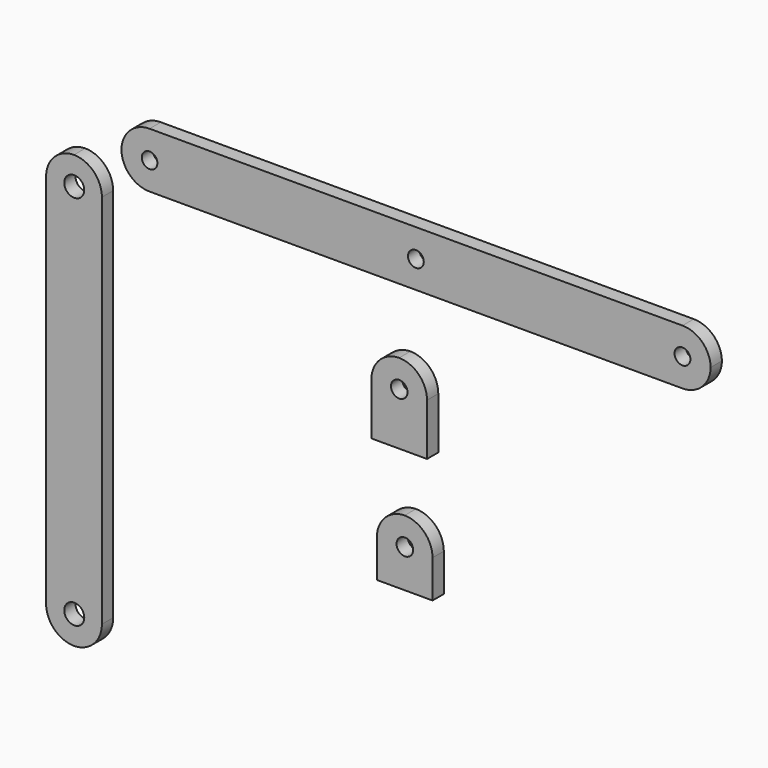
from build123d import *

# Parameters (mm, degrees)
F0_W         = 11.8872001767
F0_H         = 92.0496024191
F1_DEPTH     = 3
F2_T1_DEPTH  = 33
F3_T1_DEPTH  = 33
F4_R         = 2.1296037298
F5_DEPTH     = 25
F6_R         = 2.1316935328
F7_DEPTH     = 11.5
F8_W         = 125.4713088274
F8_H         = 11.7845982313
F9_DEPTH     = 3
F10_T1_DEPTH = 33
F11_T1_DEPTH = 33
F12_R        = 1.6622062421
F13_DEPTH    = 48.8
F14_R        = 1.68602316
F15_DEPTH    = 13.8
F16_R        = 1.68037386
F17_DEPTH    = 14.7
F18_W        = 11.8510928005
F18_H        = 17.0255154371
F19_DEPTH    = 3
F20_T1_DEPTH = 33
F21_R        = 1.75368676
F22_DEPTH    = 6.9
F23_W        = 11.8489861488
F23_H        = 14.0224687639
F24_DEPTH    = 3
F25_T1_DEPTH = 33
F26_R        = 1.7691912445
F27_DEPTH    = 16.9


# Not quite as in the source:
# - a fillet or chamfer that OpenCascade refuses, or shapes differently, is made with other operations: its cross-section is extruded or revolved along the edge and cut away or added


with BuildPart() as f1:
    # F0 (on Front) → F1 (new body)
    with BuildSketch(Plane.XZ):
        with Locations((-55.626001209, -0.7619988173)):
            Rectangle(F0_W, F0_H)
    extrude(amount=F1_DEPTH)

    # F2: fillet of radius 6 on 2 edges, made by hand

    # F2_s2 → F2_t1 (cut)
    with BuildSketch(Plane.XZ.offset(-15)):
        with BuildLine():
            ThreePointArc((-55.5696012974, 45.2628023922), (-59.8122419845, 43.5054430794), (-61.5696012974, 39.2628023922))
            Line((-61.5696012974, 39.2628023922), (-61.5696012974, 45.2628023922))
            Line((-61.5696012974, 45.2628023922), (-55.5696012974, 45.2628023922))
        make_face()
        with BuildLine():
            ThreePointArc((-55.6824011207, 45.2628023922), (-51.4397604335, 43.5054430794), (-49.6824011207, 39.2628023922))
            Line((-49.6824011207, 39.2628023922), (-49.6824011207, 45.2628023922))
            Line((-49.6824011207, 45.2628023922), (-55.6824011207, 45.2628023922))
        make_face()
    extrude(amount=F2_T1_DEPTH, mode=Mode.SUBTRACT)

    # F3: fillet of radius 6 on 2 edges, made by hand

    # F3_s2 → F3_t1 (cut)
    with BuildSketch(Plane.XZ.offset(-15)):
        with BuildLine():
            ThreePointArc((-49.6824011207, -40.7868000269), (-51.4397604335, -45.029440714), (-55.6824011207, -46.7868000269))
            Line((-55.6824011207, -46.7868000269), (-49.6824011207, -46.7868000269))
            Line((-49.6824011207, -46.7868000269), (-49.6824011207, -40.7868000269))
        make_face()
        with BuildLine():
            ThreePointArc((-55.5696012974, -46.7868000269), (-59.8122419845, -45.029440714), (-61.5696012974, -40.7868000269))
            Line((-61.5696012974, -40.7868000269), (-61.5696012974, -46.7868000269))
            Line((-61.5696012974, -46.7868000269), (-55.5696012974, -46.7868000269))
        make_face()
    extrude(amount=F3_T1_DEPTH, mode=Mode.SUBTRACT)

    # F4 (on Front) → F5 (cut)
    with BuildSketch(Plane.XZ):
        with Locations((-55.572591722, 39.3529161811)):
            Circle(F4_R)
    extrude(amount=F5_DEPTH, mode=Mode.SUBTRACT)

    # F6 (on face) → F7 (cut)
    with BuildSketch(Plane.XZ.offset(3)):
        with Locations((-55.5696012974, -40.7868000269)):
            Circle(F6_R)
    extrude(amount=-F7_DEPTH, mode=Mode.SUBTRACT)


with BuildPart() as f9:
    # F8 (on Front) → F9 (new body)
    with BuildSketch(Plane.XZ):
        with Locations((17.2029063106, 49.5063103735)):
            Rectangle(F8_W, F8_H)
    extrude(amount=F9_DEPTH)

    # F10: fillet of radius 6 on 2 edges, made by hand

    # F10_s2 → F10_t1 (cut)
    with BuildSketch(Plane.XZ.offset(-15)):
        with BuildLine():
            ThreePointArc((-39.5327481031, 55.3986094892), (-43.7753887903, 53.6412501763), (-45.5327481031, 49.3986094892))
            Line((-45.5327481031, 49.3986094892), (-45.5327481031, 55.3986094892))
            Line((-45.5327481031, 55.3986094892), (-39.5327481031, 55.3986094892))
        make_face()
        with BuildLine():
            ThreePointArc((-45.5327481031, 49.6140112579), (-43.7753887903, 45.3713705708), (-39.5327481031, 43.6140112579))
            Line((-39.5327481031, 43.6140112579), (-45.5327481031, 43.6140112579))
            Line((-45.5327481031, 43.6140112579), (-45.5327481031, 49.6140112579))
        make_face()
    extrude(amount=F10_T1_DEPTH, mode=Mode.SUBTRACT)

    # F11: fillet of radius 6 on 2 edges, made by hand

    # F11_s2 → F11_t1 (cut)
    with BuildSketch(Plane.XZ.offset(-15)):
        with BuildLine():
            ThreePointArc((73.9385607243, 55.3986094892), (78.1812014114, 53.6412501763), (79.9385607243, 49.3986094892))
            Line((79.9385607243, 49.3986094892), (79.9385607243, 55.3986094892))
            Line((79.9385607243, 55.3986094892), (73.9385607243, 55.3986094892))
        make_face()
        with BuildLine():
            ThreePointArc((79.9385607243, 49.6140112579), (78.1812014114, 45.3713705708), (73.9385607243, 43.6140112579))
            Line((73.9385607243, 43.6140112579), (79.9385607243, 43.6140112579))
            Line((79.9385607243, 43.6140112579), (79.9385607243, 49.6140112579))
        make_face()
    extrude(amount=F11_T1_DEPTH, mode=Mode.SUBTRACT)

    # F12 (on Front) → F13 (cut)
    with BuildSketch(Plane.XZ):
        with Locations((-39.5303107798, 49.4775809348)):
            Circle(F12_R)
    extrude(amount=F13_DEPTH, mode=Mode.SUBTRACT)

    # F14 (on face) → F15 (cut)
    with BuildSketch(Plane(origin=(0, 0, 0), x_dir=(-1, 0, 0), z_dir=(0, 1, 0))):
        with Locations((-73.9385607243, 49.6140112579)):
            Circle(F14_R)
    extrude(amount=-F15_DEPTH, mode=Mode.SUBTRACT)

    # F16 (on Front) → F17 (cut)
    with BuildSketch(Plane.XZ):
        with Locations((17.1728059649, 49.4200251997)):
            Circle(F16_R)
    extrude(amount=F17_DEPTH, mode=Mode.SUBTRACT)


with BuildPart() as f19:
    # F18 (on Front) → F19 (new body)
    with BuildSketch(Plane.XZ):
        with Locations((13.6170322075, 21.2140381336)):
            Rectangle(F18_W, F18_H)
    extrude(amount=F19_DEPTH)

    # F20: fillet of radius 6 on 2 edges, made by hand

    # F20_s2 → F20_t1 (cut)
    with BuildSketch(Plane.XZ.offset(-15)):
        with BuildLine():
            ThreePointArc((13.5425786078, 29.7267958522), (17.7852192949, 27.9694365393), (19.5425786078, 23.7267958522))
            Line((19.5425786078, 23.7267958522), (19.5425786078, 29.7267958522))
            Line((19.5425786078, 29.7267958522), (13.5425786078, 29.7267958522))
        make_face()
        with BuildLine():
            ThreePointArc((13.6914858073, 29.7267958522), (9.4488451202, 27.9694365393), (7.6914858073, 23.7267958522))
            Line((7.6914858073, 23.7267958522), (7.6914858073, 29.7267958522))
            Line((7.6914858073, 29.7267958522), (13.6914858073, 29.7267958522))
        make_face()
    extrude(amount=F20_T1_DEPTH, mode=Mode.SUBTRACT)

    # F21 (on Front) → F22 (cut)
    with BuildSketch(Plane.XZ):
        with Locations((13.627816923, 23.8479375839)):
            Circle(F21_R)
    extrude(amount=F22_DEPTH, mode=Mode.SUBTRACT)


with BuildPart() as f24:
    # F23 (on Front) → F24 (new body)
    with BuildSketch(Plane.XZ):
        with Locations((14.7944297642, -6.4395176305)):
            Rectangle(F23_W, F23_H)
    extrude(amount=F24_DEPTH)

    # F25: fillet of radius 6 on 2 edges, made by hand

    # F25_s2 → F25_t1 (cut)
    with BuildSketch(Plane.XZ.offset(-15)):
        with BuildLine():
            ThreePointArc((14.8699366897, 0.5717167514), (10.6272960026, -1.1856425614), (8.8699366897, -5.4282832486))
            Line((8.8699366897, -5.4282832486), (8.8699366897, 0.5717167514))
            Line((8.8699366897, 0.5717167514), (14.8699366897, 0.5717167514))
        make_face()
        with BuildLine():
            ThreePointArc((20.7189228386, -5.4282832486), (18.9615635257, -1.1856425614), (14.7189228386, 0.5717167514))
            Line((14.7189228386, 0.5717167514), (20.7189228386, 0.5717167514))
            Line((20.7189228386, 0.5717167514), (20.7189228386, -5.4282832486))
        make_face()
    extrude(amount=F25_T1_DEPTH, mode=Mode.SUBTRACT)

    # F26 (on Front) → F27 (cut)
    with BuildSketch(Plane.XZ):
        with Locations((14.828084968, -5.3094546311)):
            Circle(F26_R)
    extrude(amount=F27_DEPTH, mode=Mode.SUBTRACT)


solid = Compound([f1.part, f9.part, f19.part, f24.part])
